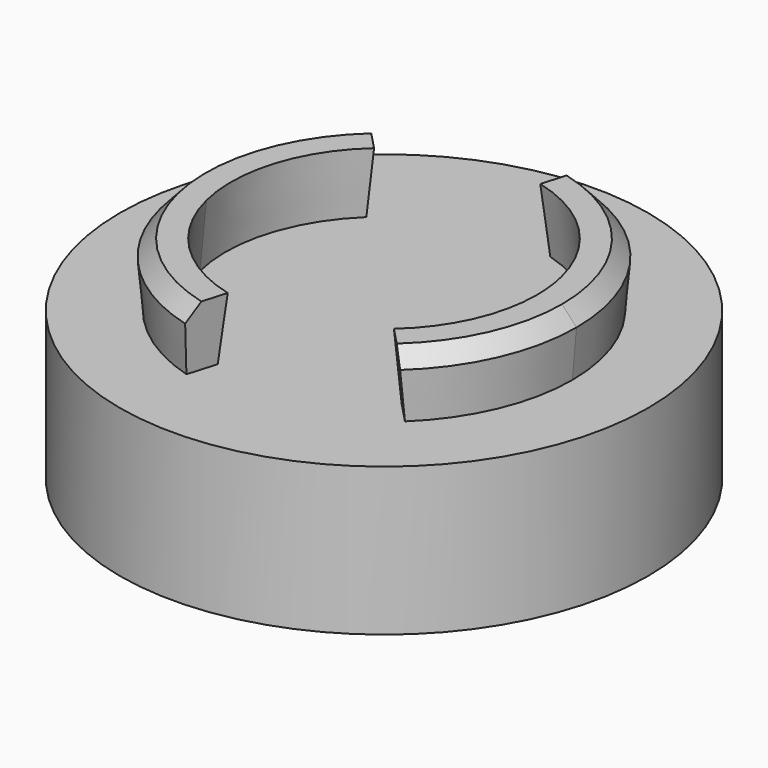
from build123d import *

# Parameters (mm, degrees)
F0_R                     = 12.5
F0_R_2                   = 8.6
F0_R_3                   = 7.5
F1_DEPTH                 = 7
F3_DEPTH                 = 3
DRAFT_F3_DRAFTED_ANGLE   = -5
DRAFT_F3_2_DRAFTED_ANGLE = -5
F4_SIZE                  = 0.75


# Not quite as in the source:
# - an extrude with a draft is written as a straight extrude whose walls are then drafted


with BuildPart() as f1:
    # F0 (on Top) → F1 (new body)
    with BuildSketch(Plane.XY):
        Circle(F0_R)
        Circle(F0_R_2, mode=Mode.SUBTRACT)
        Circle(F0_R_2)
        Circle(F0_R_3, mode=Mode.SUBTRACT)
        Circle(F0_R_3)
    extrude(amount=-F1_DEPTH)


with BuildPart() as f3_drafted:
    # F2 (on face) → F3 (new body)
    with BuildSketch(Plane.XY):
        with BuildLine():
            ThreePointArc((-8.6608975274, -2.1025946002), (-6.4492599782, -6.1513491013), (-2.5095484261, -8.5518545784))
            Line((-2.5095484261, -8.5518545784), (-2.111830016, -7.1965390281))
            ThreePointArc((-2.111830016, -7.1965390281), (-5.4271679564, -5.1764706097), (-7.2883006257, -1.7693710717))
            Line((-7.2883006257, -1.7693710717), (-8.6608975274, -2.1025946002))
        make_face()
        with BuildLine():
            Line((-5.1764706097, 5.4271679564), (-6.1513491013, 6.4492599782))
            ThreePointArc((-6.1513491013, 6.4492599782), (-8.5518545784, 2.5095484261), (-8.6608975274, -2.1025946002))
            Line((-8.6608975274, -2.1025946002), (-7.2883006257, -1.7693710717))
            ThreePointArc((-7.2883006257, -1.7693710717), (-7.1965390281, 2.111830016), (-5.1764706097, 5.4271679564))
        make_face()
    extrude(amount=F3_DEPTH)

    # draft_F3_drafted
    draft_f3_drafted_walls = [f3_drafted.faces().sort_by_distance(p)[0] for p in [
        (-7.2883006257, -1.7693710717, 2),
        (-5.6639098555, 5.9382139673, 2),
        (-8.6608975274, -2.1025946002, 2),
        (-2.310689221, -7.8741968033, 2),
    ]]
    draft(draft_f3_drafted_walls, neutral_plane=Plane.XY, angle=DRAFT_F3_DRAFTED_ANGLE)


with BuildPart() as f1_1:
    add(f1.part)

    # join_F3_drafted: union F3_drafted
    add(f3_drafted.part)


with BuildPart() as f3_2_drafted:
    # F2 (on face) → F3, piece 2 (new body)
    with BuildSketch(Plane.XY):
        with BuildLine():
            ThreePointArc((6.1513491013, -6.4492599782), (8.1931599428, -3.5077314871), (8.9124659906, 0))
            ThreePointArc((8.9124659906, 0), (7.1343645489, 5.3416189041), (2.5095484261, 8.5518545784))
            Line((2.5095484261, 8.5518545784), (2.111830016, 7.1965390281))
            ThreePointArc((2.111830016, 7.1965390281), (5.4304380841, 5.1730399394), (7.2905310718, 1.7601581439))
            ThreePointArc((7.2905310718, 1.7601581439), (7.4474486584, 0.8862891632), (7.5, 0))
            ThreePointArc((7.5, 0), (6.8946910581, -2.951818967), (5.1764706097, -5.4271679564))
            Line((5.1764706097, -5.4271679564), (6.1513491013, -6.4492599782))
        make_face()
    extrude(amount=F3_DEPTH)

    # draft_F3_2_drafted
    draft_f3_2_drafted_walls = [f3_2_drafted.faces().sort_by_distance(p)[0] for p in [
        (5.6639098555, -5.9382139673, 2),
        (2.310689221, 7.8741968033, 2),
        (8.6608975274, 2.1025946002, 2),
        (7.2883006257, 1.7693710717, 2),
    ]]
    draft(draft_f3_2_drafted_walls, neutral_plane=Plane.XY, angle=DRAFT_F3_2_DRAFTED_ANGLE)


with BuildPart() as f1_2:
    add(f1_1.part)

    # join_F3_2_drafted: union F3_2_drafted
    add(f3_2_drafted.part)

    # F4
    f4_edges = [f1_2.edges().sort_by_distance(p)[0] for p in [
        (-8.915955, -2.164515, 3),
        (8.915955, 2.164515, 3),
    ]]
    chamfer(f4_edges, length=F4_SIZE)


solid = f1_2.part
